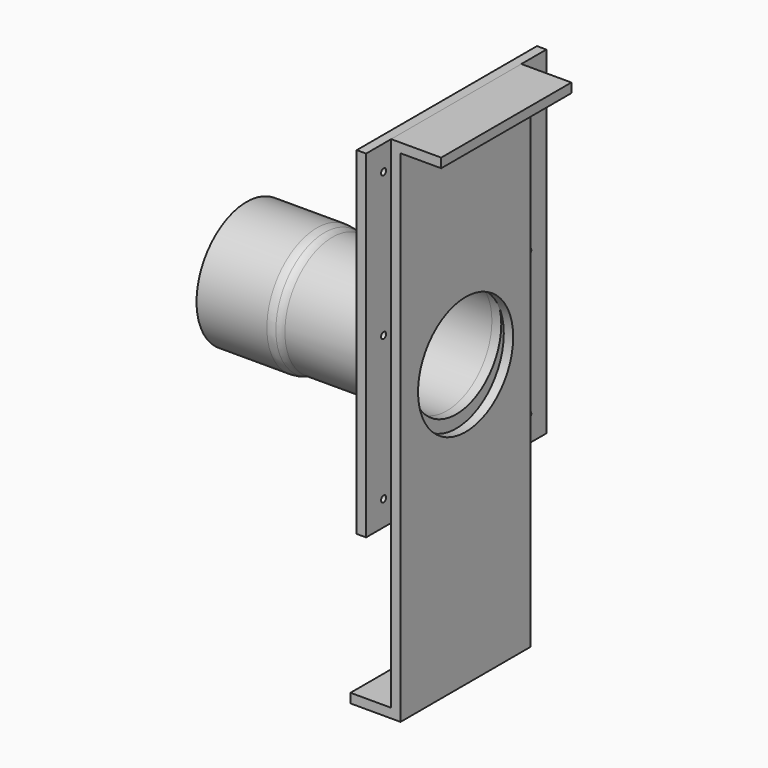
from build123d import *

# Parameters (mm, degrees)
F4_R      = 10.16
F5_W      = 114.3
F5_H      = 171.45
F6_DEPTH  = 4.7625
F7_DEPTH  = 4.7635
F8_R      = 1.5875
F9_DEPTH  = 106.3635001
F11_DEPTH = 41.275
F12_R     = 30.1625
F13_DEPTH = 111.1260001


# Not quite as in the source:
# - a fillet or chamfer that OpenCascade refuses, or shapes differently, is made with other operations: its cross-section is extruded or revolved along the edge and cut away or added
# - a pattern or mirror of a feature is missing from the dataset's text; its kind, count and spacing are read off the source's solid


with BuildPart() as f2:
    # F0 (on Top) → F2 (revolve)
    with BuildSketch(Plane.XY):
        Polygon((-65.0875, 28.575), (0, 28.575), (0, 30.1625), (-63.5, 30.1625), (-63.5, 31.75), (-101.6, 31.75), (-101.6, 30.1625), (-65.0875, 30.1625), align=None)
    revolve(axis=Axis((-31.0941394418, 0, 0), (-1, 0, 0)))

    # F3: fillet of radius 10.16 on 1 edges, made by hand

    # F3_s1 → F3_t2 (revolve)
    with BuildSketch(Plane.XY):
        with BuildLine():
            ThreePointArc((-58.0467584182, 30.1625), (-60.8865647496, 30.5674449002), (-63.5, 31.75))
            Line((-63.5, 31.75), (-63.5, 30.1625))
            Line((-63.5, 30.1625), (-58.0467584182, 30.1625))
        make_face()
    revolve(axis=Axis((-63.5, 0, 0), (-1, 0, 0)))

    # F4
    f4_edges = [f2.edges().sort_by_distance(p)[0] for p in [
        (-63.5, -31.75, 0),
    ]]
    fillet(f4_edges, radius=F4_R)

    # F5 (on Right) → F6 (join)
    with BuildSketch(Plane.YZ):
        with Locations((0, 25.4)):
            Rectangle(F5_W, F5_H)
    extrude(amount=F6_DEPTH)

    # F7 (cut, through all): a face of the model
    f7_faces = [f2.faces().sort_by_distance(p)[0] for p in [
        (0, 0, 0),
    ]]
    extrude(f7_faces, amount=-F7_DEPTH, mode=Mode.SUBTRACT)

    # F8 (on face) → F9 (cut, through all)
    with BuildSketch(Plane.YZ.offset(4.7625)):
        with Locations((-46.0375, -47.625)):
            Circle(F8_R)
        with Locations((-46.0375, 25.4)):
            Circle(F8_R)
        with Locations((-46.0375, 98.425)):
            Circle(F8_R)
    f9 = extrude(amount=-F9_DEPTH, mode=Mode.SUBTRACT)

    # F9_copies: F9 across plane
    add(f9.mirror(Plane.ZX), mode=Mode.SUBTRACT)


with BuildPart() as f11:
    # F10 (on Front) → F11 (new body, symmetric)
    with BuildSketch(Plane.XZ):
        Polygon((4.7625, 111.125), (4.7625, -142.875), (-15.875, -142.875), (-15.875, -147.6375), (9.525, -147.6375), (9.525, 106.3625), (30.1625, 106.3625), (30.1625, 111.125), align=None)
    extrude(amount=F11_DEPTH, both=True)

    # F12 (on face) → F13 (cut, through all)
    with BuildSketch(Plane.YZ.offset(9.525)):
        with Locations((0, -4.7625)):
            Circle(F12_R)
    extrude(amount=-F13_DEPTH, mode=Mode.SUBTRACT)


solid = Compound([f2.part, f11.part])
